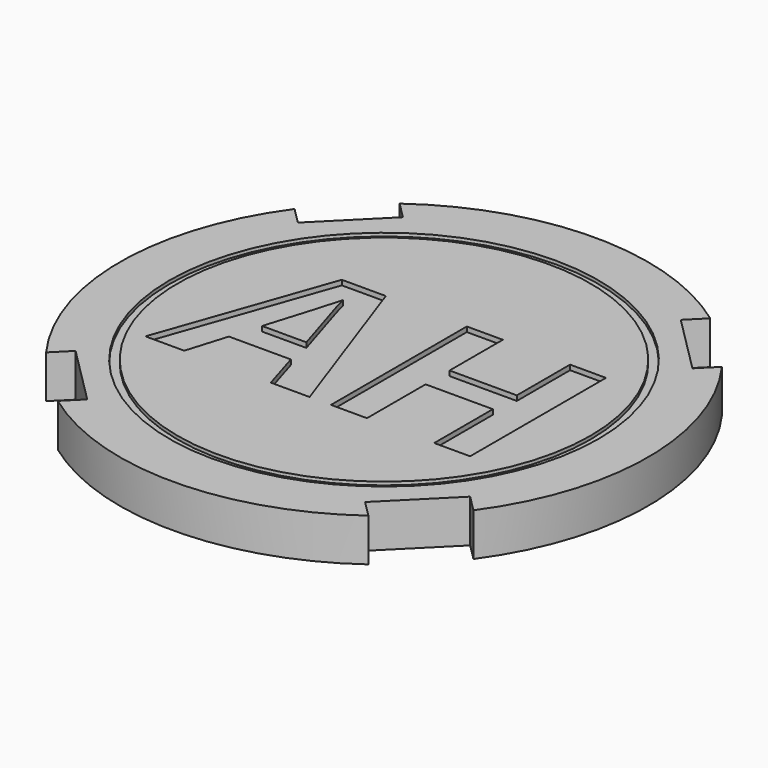
from build123d import *

# Parameters (mm, degrees)
F0_R          = 20.32
F1_DEPTH      = 3.302
F6_DEPTH      = 3.302
F7_R          = 16.51
F7_R_2        = 15.875
F8_DEPTH      = 0.254
F2_TEXT_SIZE  = 8.7192824304
F9_DEPTH      = 0.381
F3_TEXT_SIZE  = 8.8355448193
F10_DEPTH     = 0.381
F4_TEXT_SIZE  = 6.4111328842
F11_DEPTH     = 0.381
F12_TEXT_SIZE = 18.2991038251
F13_DEPTH     = 0.381


# Not quite as in the source:
# - Text() gives the source's letters only with a copy of the font that has no kerning and outlines rounded to 1/6400 em; it was checked with that copy


with BuildPart() as f1:
    # F0 (on Top) → F1 (new body)
    with BuildSketch(Plane.XY):
        Circle(F0_R)
    extrude(amount=F1_DEPTH)

    # F5 (on face) → F6 (cut)
    with BuildSketch(Plane(origin=(0, 0, 0), x_dir=(1, 0, 0), z_dir=(0, 0, -1))):
        with BuildLine():
            Line((-16.4369943958, 11.9468663353), (-15.1766328446, 10.6865047841))
            Line((-15.1766328446, 10.6865047841), (-10.6865047841, 15.1766328446))
            Line((-10.6865047841, 15.1766328446), (-11.9468663353, 16.4369943958))
            ThreePointArc((-11.9468663353, 16.4369943958), (-14.3684097937, 14.3684097937), (-16.4369943958, 11.9468663353))
        make_face()
        with BuildLine():
            Line((-10.6865047841, -15.1766328446), (-15.1766328446, -10.6865047841))
            Line((-15.1766328446, -10.6865047841), (-16.4369943958, -11.9468663353))
            ThreePointArc((-16.4369943958, -11.9468663353), (-14.3684097937, -14.3684097937), (-11.9468663353, -16.4369943958))
            Line((-11.9468663353, -16.4369943958), (-10.6865047841, -15.1766328446))
        make_face()
        with BuildLine():
            Line((15.1766328446, -10.6865047841), (10.6865047841, -15.1766328446))
            Line((10.6865047841, -15.1766328446), (11.9468663353, -16.4369943958))
            ThreePointArc((11.9468663353, -16.4369943958), (14.3684097937, -14.3684097937), (16.4369943958, -11.9468663353))
            Line((16.4369943958, -11.9468663353), (15.1766328446, -10.6865047841))
        make_face()
        with BuildLine():
            Line((10.6865047841, 15.1766328446), (15.1766328446, 10.6865047841))
            Line((15.1766328446, 10.6865047841), (16.4369943958, 11.9468663353))
            ThreePointArc((16.4369943958, 11.9468663353), (14.3684097937, 14.3684097937), (11.9468663353, 16.4369943958))
            Line((11.9468663353, 16.4369943958), (10.6865047841, 15.1766328446))
        make_face()
    extrude(amount=-F6_DEPTH, mode=Mode.SUBTRACT)

    # F7 (on face) → F8 (cut)
    with BuildSketch(Plane.XY.offset(3.302)):
        Circle(F7_R)
        Circle(F7_R_2, mode=Mode.SUBTRACT)
    extrude(amount=-F8_DEPTH, mode=Mode.SUBTRACT)

    # F2 (on face) → F9 (cut)
    with BuildSketch(Plane(origin=(0, 0, 0), x_dir=(1, 0, 0), z_dir=(0, 0, -1))):
        with Locations((-19.4460434017, -3.138941675)):
            Text('Bachelor', F2_TEXT_SIZE, font='Open Sans', font_style=FontStyle.BOLD, text_align=(TextAlign.LEFT, TextAlign.BOTTOM))
    extrude(amount=-F9_DEPTH, mode=Mode.SUBTRACT)

    # F3 (on face) → F10 (cut)
    with BuildSketch(Plane(origin=(0, 0, 0), x_dir=(1, 0, 0), z_dir=(0, 0, -1))):
        with Locations((-8.001, 8.218941675)):
            Text("AJ's", F3_TEXT_SIZE, font='Open Sans', font_style=FontStyle.BOLD, text_align=(TextAlign.LEFT, TextAlign.BOTTOM))
    extrude(amount=-F10_DEPTH, mode=Mode.SUBTRACT)

    # F4 (on face) → F11 (cut)
    with BuildSketch(Plane(origin=(0, 0, 0), x_dir=(1, 0, 0), z_dir=(0, 0, -1))):
        with Locations((-8.8278294597, -12.8349573516)):
            Text('Party', F4_TEXT_SIZE, font='Open Sans', font_style=FontStyle.BOLD, text_align=(TextAlign.LEFT, TextAlign.BOTTOM))
    extrude(amount=-F11_DEPTH, mode=Mode.SUBTRACT)

    # F12 (on face) → F13 (cut)
    with BuildSketch(Plane.XY.offset(3.302)):
        with Locations((-13.081, -6.587677377)):
            Text('AH', F12_TEXT_SIZE, font='Open Sans', font_style=FontStyle.BOLD, text_align=(TextAlign.LEFT, TextAlign.BOTTOM))
    extrude(amount=-F13_DEPTH, mode=Mode.SUBTRACT)


solid = f1.part
